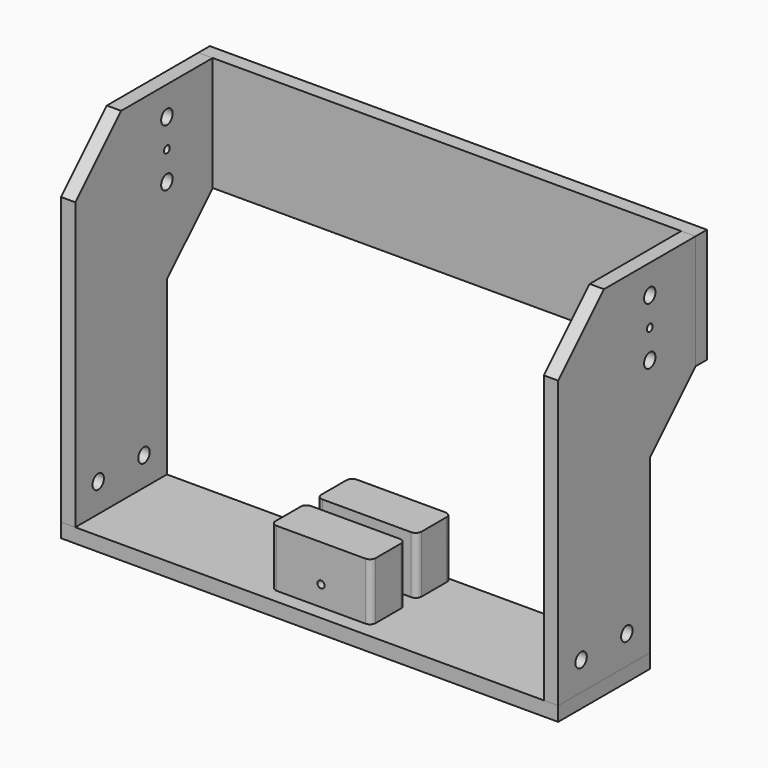
from build123d import *

# Parameters (mm, degrees)
F0_W      = 50.8
F0_H      = 101.6
F1_DEPTH  = 12.7
F2_W      = 101.6
F2_H      = 12.7
F3_DEPTH  = 441.325
F4_R      = 6.35
F4_R_2    = 3.175
F5_DEPTH  = 25.4
F8_W      = 12.7
F8_H      = 101.6
F9_DEPTH  = 441.325
F11_DEPTH = 508
F12_W     = 88.9
F12_H     = 38.1
F13_DEPTH = 50.8
F14_R     = 5.08
F14_2_R   = 5.08
F15_R     = 2.8575
F16_DEPTH = 25.4
F17_R     = 3.175
F18_DEPTH = 101.6
F19_R     = 2.8575
F20_DEPTH = 38.1
F21_R     = 2.8575
F22_DEPTH = 38.1


# Not quite as in the source:
# - a feature names something its author has since deleted; it is built from what else it names


with BuildPart() as f1:
    # F0 (on Right) → F1 (new body)
    with BuildSketch(Plane.YZ):
        Polygon((50.8, 50.8), (-50.8, 50.8), (-50.8, -152.4), (50.8, -152.4), (50.8, 0), align=None)
        with Locations((76.2, 101.6)):
            Rectangle(F0_W, F0_H)
        Polygon((50.8, 152.4), (0, 152.4), (-50.8, 101.6), (-50.8, 50.8), (50.8, 50.8), align=None)
        Polygon((101.6, 50.8), (50.8, 50.8), (50.8, 0), align=None)
    extrude(amount=F1_DEPTH)

    # F4 (on face) → F5 (cut)
    with BuildSketch(Plane.YZ.offset(12.7)):
        with Locations((50.8, 127)):
            Circle(F4_R)
        with Locations((50.8, 101.6)):
            Circle(F4_R_2)
        with Locations((50.8, 76.2)):
            Circle(F4_R)
    extrude(amount=-F5_DEPTH, mode=Mode.SUBTRACT)


with BuildPart() as f3:
    # F2 (on Right) → F3 (new body)
    with BuildSketch(Plane.YZ):
        with Locations((0, -158.75)):
            Rectangle(F2_W, F2_H)
    extrude(amount=F3_DEPTH)


with BuildPart() as f7_1:
    # F7: instance of F1
    add(f1.part.mirror(Plane.YZ.offset(220.6625)))


with BuildPart() as f9:
    # F8 (on Right) → F9 (new body)
    with BuildSketch(Plane.YZ):
        with Locations((107.95, 101.6)):
            Rectangle(F8_W, F8_H)
    extrude(amount=F9_DEPTH)


with BuildPart() as f11_tool:
    # F10 (on face) → F11 (new body)
    with BuildSketch(Plane.YZ.offset(441.325)):
        with BuildLine():
            Line((-25.4, -127), (-19.05, -127))
            ThreePointArc((-19.05, -127), (-25.4, -120.65), (-31.75, -127))
            Line((-31.75, -127), (-25.4, -127))
        make_face()
        with BuildLine():
            ThreePointArc((-31.75, -127), (-25.4, -133.35), (-19.05, -127))
            Line((-19.05, -127), (-25.4, -127))
            Line((-25.4, -127), (-31.75, -127))
        make_face()
        with BuildLine():
            ThreePointArc((31.75, -127), (25.4, -120.65), (19.05, -127))
            Line((19.05, -127), (25.4, -127))
            Line((25.4, -127), (31.75, -127))
        make_face()
        with BuildLine():
            Line((25.4, -127), (19.05, -127))
            ThreePointArc((19.05, -127), (25.4, -133.35), (31.75, -127))
            Line((31.75, -127), (25.4, -127))
        make_face()
    extrude(amount=-F11_DEPTH)


with BuildPart() as f1_1:
    add(f1.part)

    # F11: cut by f11_tool
    add(f11_tool.part, mode=Mode.SUBTRACT)


with BuildPart() as f7_1_1:
    add(f7_1.part)

    # F11: cut by f11_tool
    add(f11_tool.part, mode=Mode.SUBTRACT)


with BuildPart() as f13:
    # F12 (on face) → F13 (new body)
    with BuildSketch(Plane.XY.offset(-152.4)):
        with Locations((220.6625, -19.05)):
            Rectangle(F12_W, F12_H)
    extrude(amount=F13_DEPTH)

    # F14
    f14_edges = [f13.edges().sort_by_distance(p)[0] for p in [
        (176.2125, -38.1, -127),
        (176.2125, 0, -127),
        (265.1125, -38.1, -127),
        (265.1125, 0, -127),
    ]]
    fillet(f14_edges, radius=F14_R)


with BuildPart() as f13b:
    # F12 (on face) → F13, piece 2 (new body)
    with BuildSketch(Plane.XY.offset(-152.4)):
        with Locations((220.6625, 31.75)):
            Rectangle(F12_W, F12_H)
    extrude(amount=F13_DEPTH)

    # F14#2
    f14_2_edges = [f13b.edges().sort_by_distance(p)[0] for p in [
        (176.2125, 12.7, -127),
        (265.1125, 12.7, -127),
        (265.1125, 50.8, -127),
        (176.2125, 50.8, -127),
    ]]
    fillet(f14_2_edges, radius=F14_2_R)


with BuildPart() as f16_tool:
    # F15 (on face) → F16 (new body)
    with BuildSketch(Plane(origin=(0, 0, -165.1), x_dir=(1, 0, 0), z_dir=(0, 0, -1))):
        with Locations((195.2625, 19.05)):
            Circle(F15_R)
        with Locations((246.0625, 19.05)):
            Circle(F15_R)
        with Locations((195.2625, -31.75)):
            Circle(F15_R)
        with Locations((246.0625, -31.75)):
            Circle(F15_R)
    extrude(amount=-F16_DEPTH)


with BuildPart() as f3_1:
    add(f3.part)

    # F16: cut by f16_tool
    add(f16_tool.part, mode=Mode.SUBTRACT)

    # F21 (on face) → F22 (cut)
    with BuildSketch(Plane(origin=(0, 0, -165.1), x_dir=(1, 0, 0), z_dir=(0, 0, -1))):
        with Locations((195.2625, 19.05)):
            Circle(F21_R)
        with Locations((246.0625, 19.05)):
            Circle(F21_R)
        with Locations((195.2625, -31.75)):
            Circle(F21_R)
        with Locations((246.0625, -31.75)):
            Circle(F21_R)
        with BuildLine():
            Line((434.975, 22.5425), (434.975, 28.2575))
            ThreePointArc((434.975, 28.2575), (432.1175, 25.4), (434.975, 22.5425))
        make_face()
        with BuildLine():
            ThreePointArc((437.8325, 25.4), (436.9955576272, 27.4205576272), (434.975, 28.2575))
            Line((434.975, 28.2575), (434.975, 22.5425))
            ThreePointArc((434.975, 22.5425), (436.9955576272, 23.3794423728), (437.8325, 25.4))
        make_face()
        with BuildLine():
            Line((434.975, -28.2575), (434.975, -22.5425))
            ThreePointArc((434.975, -22.5425), (432.1175, -25.4), (434.975, -28.2575))
        make_face()
        with BuildLine():
            ThreePointArc((437.8325, -25.4), (436.9955576272, -23.3794423728), (434.975, -22.5425))
            Line((434.975, -22.5425), (434.975, -28.2575))
            ThreePointArc((434.975, -28.2575), (436.9955576272, -27.4205576272), (437.8325, -25.4))
        make_face()
        with BuildLine():
            Line((6.35, -28.2575), (6.35, -22.5425))
            ThreePointArc((6.35, -22.5425), (3.4925, -25.4), (6.35, -28.2575))
        make_face()
        with BuildLine():
            ThreePointArc((9.2075, -25.4), (8.3705576272, -23.3794423728), (6.35, -22.5425))
            Line((6.35, -22.5425), (6.35, -28.2575))
            ThreePointArc((6.35, -28.2575), (8.3705576272, -27.4205576272), (9.2075, -25.4))
        make_face()
        with BuildLine():
            Line((6.35, 22.5425), (6.35, 28.2575))
            ThreePointArc((6.35, 28.2575), (3.4925, 25.4), (6.35, 22.5425))
        make_face()
        with BuildLine():
            ThreePointArc((9.2075, 25.4), (8.3705576272, 27.4205576272), (6.35, 28.2575))
            Line((6.35, 28.2575), (6.35, 22.5425))
            ThreePointArc((6.35, 22.5425), (8.3705576272, 23.3794423728), (9.2075, 25.4))
        make_face()
    extrude(amount=-F22_DEPTH, mode=Mode.SUBTRACT)


with BuildPart() as f13_1:
    add(f13.part)

    # F16: cut by f16_tool
    add(f16_tool.part, mode=Mode.SUBTRACT)


with BuildPart() as f13b_1:
    add(f13b.part)

    # F16: cut by f16_tool
    add(f16_tool.part, mode=Mode.SUBTRACT)


with BuildPart() as f18_tool:
    # F17 (on face) → F18 (new body)
    with BuildSketch(Plane.XZ.offset(38.1)):
        with Locations((220.6615805626, -134.62)):
            Circle(F17_R)
    extrude(amount=-F18_DEPTH)


with BuildPart() as f13_2:
    add(f13_1.part)

    # F18: cut by f18_tool
    add(f18_tool.part, mode=Mode.SUBTRACT)


with BuildPart() as f13b_2:
    add(f13b_1.part)

    # F18: cut by f18_tool
    add(f18_tool.part, mode=Mode.SUBTRACT)


with BuildPart() as f20_tool:
    # F19 (on face) → F20 (new body)
    with BuildSketch(Plane(origin=(0, 114.3, 0), x_dir=(-1, 0, 0), z_dir=(0, 1, 0))):
        with Locations((-6.35, 133.35)):
            Circle(F19_R)
        with Locations((-6.35, 69.85)):
            Circle(F19_R)
        with Locations((-434.975, 133.35)):
            Circle(F19_R)
        with Locations((-434.975, 69.85)):
            Circle(F19_R)
    extrude(amount=-F20_DEPTH)


with BuildPart() as f1_2:
    add(f1_1.part)

    # F20: cut by f20_tool
    add(f20_tool.part, mode=Mode.SUBTRACT)


with BuildPart() as f7_1_2:
    add(f7_1_1.part)

    # F20: cut by f20_tool
    add(f20_tool.part, mode=Mode.SUBTRACT)


with BuildPart() as f9_1:
    add(f9.part)

    # F20: cut by f20_tool
    add(f20_tool.part, mode=Mode.SUBTRACT)


solid = Compound([f3_1.part, f13_2.part, f13b_2.part, f1_2.part, f7_1_2.part, f9_1.part])
